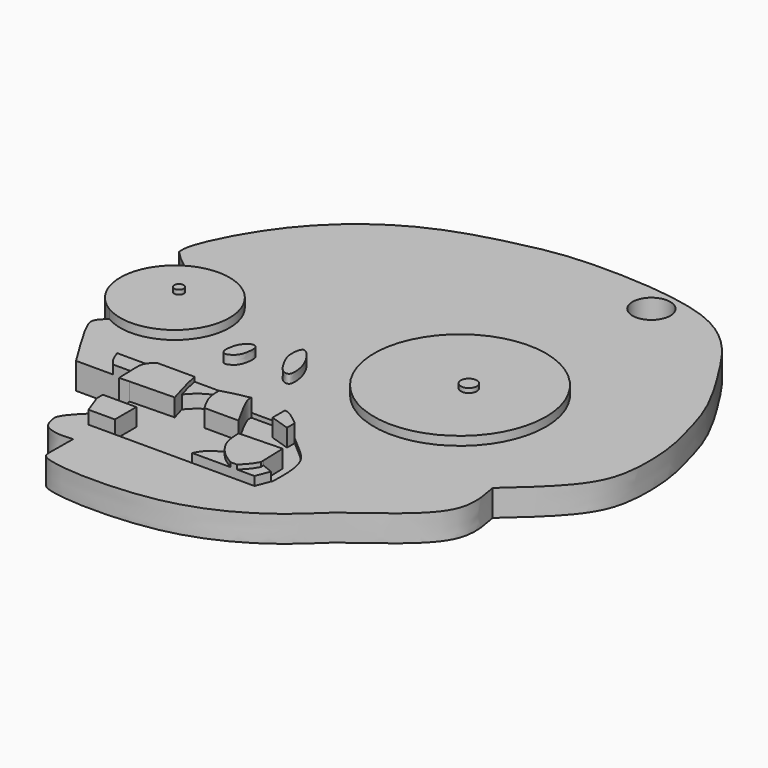
from build123d import *

# Parameters (mm, degrees)
F0_R     = 9.756
F0_R_2   = 2.14301661
F1_DEPTH = 3
F0_R_3   = 0.5489550531
F0_R_4   = 0.9110758453
F2_DEPTH = 4
F3_DEPTH = 4.5
F4_DEPTH = 4.5
F5_DEPTH = 2.5


# Not quite as in the source:
# - ends of sketch curves that miss each other by under 0.0002 mm in the source are joined


with BuildPart() as f1:
    # F0 (on Top) → F1 (new body)
    with BuildSketch(Plane.XY):
        with BuildLine():
            add(Edge.make_bspline(
                [(-1.2393802172, 30.2286203951), (-0.4158833716, 30.373480778), (1.6606665352, 30.7387642837), (7.9386116813, 30.9430876865), (18.147479825, 29.9352400746), (23.1024202655, 25.7119331789), (25.72137538, 21.6124660135), (29.4314571956, 15.6799496131), (30.7334478805, 10.40848904), (31.4866231448, 7.6721319387), (31.7667483963, 2.2460729415), (30.3960792989, -2.5468600017), (26.2945647642, -6.1923512069), (23.9523444325, -8.2741538063)],
                knots=[0, 0, 0, 0, 0.0633267686, 0.1596863377, 0.2826691674, 0.3774808941, 0.4616409818, 0.5634971311, 0.6515777447, 0.7163703966, 0.8033752015, 0.8877149899, 1, 1, 1, 1], degree=3))
            add(Edge.make_bspline(
                [(-1.2393802172, 30.2286203951), (-2.8705070942, 29.8823566818), (-6.4988427986, 29.112115561), (-14.107033655, 26.5390353225), (-22.1790734534, 19.7802047992), (-26.231732067, 11.4546819847), (-26.1231331955, 10.1430820977), (-26.0920431465, 9.7675928846)],
                knots=[0, 0, 0, 0, 0.1823196445, 0.4055581972, 0.6703764425, 0.9056342628, 1, 1, 1, 1], degree=3))
            add(Edge.make_bspline(
                [(-26.0920431465, 9.7675928846), (-25.7886867903, 9.446402666), (-25.0293246752, 8.6417283139), (-23.384300951, 7.4507044648), (-22.3954650109, 6.7330964966)],
                knots=[0, 0, 0, 0, 0.3993621606, 1, 1, 1, 1], degree=3))
            ThreePointArc((-22.3954650109, 6.7330964966), (-16.388075709, 6.4168152727), (-13.4720232753, 1.1551236967))
            ThreePointArc((-13.4720232753, 1.1551236967), (-16.6204187962, -4.2448565962), (-22.8706838798, -4.1650574556))
            add(Edge.make_bspline(
                [(-22.8706838798, -4.1650574556), (-23.2251432704, -4.503107188), (-23.8543858706, -5.1018227163), (-23.8274706305, -6.1029660819), (-22.5427366396, -8.3753891262), (-20.3011528826, -12.0943672024), (-20.1644091369, -12.2649352771), (-20.1410669833, -12.2940531)],
                knots=[0, 0, 0, 0, 0.1843482912, 0.3279717022, 0.5995926127, 0.9316769819, 1, 1, 1, 1], degree=3))
            Line((-20.1410669833, -12.2940531), (-15.9410070627, -12.2940531))
            add(Edge.make_bspline(
                [(-15.9410070627, -12.2940531), (-16.1547290947, -12.0513152103), (-16.6081258621, -11.5363632725), (-16.8757984305, -10.7686429845), (-17.0172955841, -10.3628104553)],
                knots=[0, 0, 0, 0, 0.4713796997, 1, 1, 1, 1], degree=3))
            Line((-17.0172955841, -10.3628104553), (-12.5004155561, -10.3628104553))
            Line((-12.5004155561, -10.3628104553), (-8.2129081711, -10.3628104553))
            Line((-8.2129081711, -10.3628104553), (-1.7728252569, -10.3628104553))
            Line((-1.7728252569, -10.3628104553), (1.3264130102, -10.3628104553))
            add(Edge.make_bspline(
                [(1.3264130102, -10.3628104553), (1.5699030442, -10.3549216682), (1.8133930781, -10.3470328812), (2.068254631, -10.389211361)],
                knots=[0, 0, 0, 0, 0.2797726741, 0.2797726741, 0.2797726741, 0.2797726741], degree=3))
            add(Edge.make_bspline(
                [(2.068254631, -10.389211361), (2.1914664058, -10.4096023744), (2.8617166916, -10.580494915), (3.6437610552, -11.2436017254), (4.2789415456, -11.7821805179)],
                knots=[0.2797726741, 0.2797726741, 0.2797726741, 0.2797726741, 0.4150276285, 1, 1, 1, 1], degree=3))
            add(Edge.make_bspline(
                [(4.2789415456, -11.7821805179), (4.6829303138, -12.1450168981), (5.5999948022, -12.9686644486), (8.0560238989, -14.8958762571), (7.9619883229, -17.9183800715), (7.9091731459, -19.6159724146)],
                knots=[0, 0, 0, 0, 0.2565884637, 0.5824621541, 1, 1, 1, 1], degree=3))
            add(Edge.make_bspline(
                [(7.8397894075, -19.5867830955), (7.8639386907, -19.5968842625), (7.8865559183, -19.6064283386), (7.9091731459, -19.6159724146)],
                knots=[0.8931074225, 0.8931074225, 0.8931074225, 0.8931074225, 1, 1, 1, 1], degree=3))
            add(Edge.make_bspline(
                [(7.2210850194, -21.1771205068), (7.4273304113, -20.6469827043), (7.6335758032, -20.1168449019), (7.8397894075, -19.5867830955)],
                knots=[0, 0, 0, 0, 1.7065313537, 1.7065313537, 1.7065313537, 1.7065313537], degree=3))
            Line((7.2210850194, -21.1771205068), (5.2385437302, -21.1771205068))
            Line((5.2385437302, -21.1771205068), (4.5115393586, -21.1771205068))
            Line((4.5115393586, -21.1771205068), (0.1495117176, -21.1771205068))
            Line((0.1495117176, -21.1771205068), (-8.6269685999, -21.1771205068))
            Line((-8.6269685999, -21.1771205068), (-11.6212656721, -21.1771205068))
            Line((-11.6212656721, -21.1771205068), (-12.4197443947, -18.9932379872))
            Line((-12.4197443947, -18.9932379872), (-12.5852758065, -19.1398113966))
            add(Edge.make_bspline(
                [(-10.952696187, -24.1973703964), (-11.6003607025, -24.2475742409), (-12.8304027144, -24.3429211934), (-14.4581285949, -23.7254439522), (-14.6736070417, -22.6233199395), (-15.038550408, -21.5870552272), (-13.5615867359, -20.1137223062), (-12.5852758065, -19.1398113966)],
                knots=[0, 0, 0, 0, 0.2162457448, 0.4106931052, 0.5661826538, 0.7132355897, 1, 1, 1, 1], degree=3))
            add(Edge.make_bspline(
                [(23.9523444325, -8.2741538063), (24.2863039744, -9.9748611419), (25.0090136589, -13.6552999598), (19.3340818803, -18.3065983827), (15.7324066153, -20.7445567564), (13.2149854072, -23.5297131407), (4.0834935552, -29.8946094699), (-10.9302506494, -29.1906042728), (-11.0010002399, -27.4544620035), (-10.9523846246, -24.5344095892), (-10.9525207478, -24.2320520286), (-10.952696187, -24.1973703964)],
                knots=[0, 0, 0, 0, 0.1169433124, 0.2530727642, 0.3618233297, 0.4588114113, 0.6358882656, 0.8281973553, 0.8861964274, 0.976190375, 0.9925215819, 0.9925215819, 0.9925215819, 0.9925215819], degree=3))
        make_face()
        with BuildLine():
            add(Edge.make_bspline(
                [(-9.6221137792, -2.3781536147), (-9.4655224083, -2.0993212718), (-9.0208657927, -1.6374110115), (-8.5262366968, -1.4918482785), (-8.0548862611, -1.7768664904), (-8.0508374383, -2.8141169089), (-8.3507435947, -3.8951758217), (-9.0186010158, -4.4028924818), (-9.7088724417, -4.5819747824), (-9.9941823947, -3.9236958827), (-9.8756994925, -3.1639822237), (-9.7687938604, -2.6393375514), (-9.6221137792, -2.3781536147)],
                knots=[0, 0, 0, 0, 0.1138345197, 0.1934305742, 0.2698157261, 0.3849908147, 0.5088302527, 0.6140567508, 0.7027480415, 0.7907303024, 0.8933705191, 1, 1, 1, 1], degree=3))
        make_face(mode=Mode.SUBTRACT)
        with BuildLine():
            add(Edge.make_bspline(
                [(-4.581714049, 0.4414755676), (-4.3886019619, 0.556001698), (-3.6219717469, -0.0557970156), (-2.5850360287, -1.81802008), (-2.4065766969, -3.5191596454), (-2.627381433, -4.0742860536), (-3.5558163843, -3.9967136296), (-4.6097436694, -2.0631900411), (-4.9778002041, -1.0265364593), (-4.8177214639, 0.3015101394), (-4.581714049, 0.4414755676)],
                knots=[0, 0, 0, 0, 0.1053234474, 0.2714857478, 0.4152922703, 0.4898158762, 0.5821472357, 0.743142993, 0.8712814152, 1, 1, 1, 1], degree=3))
        make_face(mode=Mode.SUBTRACT)
        with Locations((10.5493292212, 3.8432257716)):
            Circle(F0_R, mode=Mode.SUBTRACT)
        with Locations((13.4515836835, 27.3811984807)):
            Circle(F0_R_2, mode=Mode.SUBTRACT)
    extrude(amount=F1_DEPTH)

    # F0 (on Top) → F2 (join)
    with BuildSketch(Plane.XY):
        with BuildLine():
            add(Edge.make_bspline(
                [(-15.9410070627, -12.2940531), (-16.1547290947, -12.0513152103), (-16.6081258621, -11.5363632725), (-16.8757984305, -10.7686429845), (-17.0172955841, -10.3628104553)],
                knots=[0, 0, 0, 0, 0.4713796997, 1, 1, 1, 1], degree=3))
            Line((-15.9410070627, -12.2940531), (-13.3990075059, -12.2940531))
            add(Edge.make_bspline(
                [(-12.5004155561, -10.3628104553), (-12.8042925116, -10.6364223183), (-13.3531482467, -11.1306139227), (-13.4030830888, -11.8825646099), (-13.3990075059, -12.2940531)],
                knots=[0, 0, 0, 0, 0.2822962739, 0.5098771923, 0.5098771923, 0.5098771923, 0.5098771923], degree=3))
            Line((-12.5004155561, -10.3628104553), (-17.0172955841, -10.3628104553))
        make_face()
        with BuildLine():
            Line((-1.7728252569, -10.3628104553), (-8.2129081711, -10.3628104553))
            add(Edge.make_bspline(
                [(-8.2129081711, -10.3628104553), (-8.1550609219, -10.7006143743), (-8.0476180243, -11.3280362889), (-7.747571442, -12.4158381016), (-7.5893943801, -12.9649978611)],
                knots=[0, 0, 0, 0, 0.3777900329, 0.7016903371, 0.7016903371, 0.7016903371, 0.7016903371], degree=3))
            add(Edge.make_bspline(
                [(-7.5893943801, -12.9649978611), (-7.1117267836, -12.4364258807), (-6.4364554435, -11.6928519992), (-5.2333924432, -11.2084781414), (-4.8551141513, -11.0839256667)],
                knots=[0, 0, 0, 0, 0.4202161524, 0.5907091248, 0.5907091248, 0.5907091248, 0.5907091248], degree=3))
            add(Edge.make_bspline(
                [(-4.8551141513, -11.0839256667), (-3.9470072013, -10.7849210176), (-2.8599860204, -10.5738001088), (-1.7728252569, -10.3628104553)],
                knots=[0.5907091248, 0.5907091248, 0.5907091248, 0.5907091248, 1, 1, 1, 1], degree=3))
        make_face()
        with BuildLine():
            add(Edge.make_bspline(
                [(2.2680953621, -19.1644323351), (1.7322527396, -19.4720374585), (0.7474409463, -20.0374812634), (0.3369805018, -20.819646162), (0.1495117176, -21.1771205068)],
                knots=[0, 0, 0, 0, 0.5430655229, 1, 1, 1, 1], degree=3))
            Line((0.1495117176, -21.1771205068), (4.5115393586, -21.1771205068))
            add(Edge.make_bspline(
                [(2.2680953621, -19.1644323351), (2.5004401266, -19.5374508957), (3.2173678001, -20.3983675028), (4.0257518369, -20.8848033952), (4.5115393586, -21.1771205068)],
                knots=[0.4760539781, 0.4760539781, 0.4760539781, 0.4760539781, 0.6851416803, 1, 1, 1, 1], degree=3))
        make_face()
        with BuildLine():
            add(Edge.make_bspline(
                [(6.5981289918, -19.4641191504), (6.4561431042, -19.7211838775), (6.1459175946, -20.2828455842), (5.5575977759, -20.8626723579), (5.2385437302, -21.1771205068)],
                knots=[0, 0, 0, 0, 0.4576860484, 1, 1, 1, 1], degree=3))
            Line((5.2385437302, -21.1771205068), (7.2210850194, -21.1771205068))
            add(Edge.make_bspline(
                [(7.2210850194, -21.1771205068), (7.4273304113, -20.6469827043), (7.6335758032, -20.1168449019), (7.8398211952, -19.5867070995)],
                knots=[0, 0, 0, 0, 1.7065313537, 1.7065313537, 1.7065313537, 1.7065313537], degree=3))
            add(Edge.make_bspline(
                [(6.5868723652, -19.0981086926), (7.0054958994, -19.2586307437), (7.5616668588, -19.4718956366), (7.7898889474, -19.5659107211), (7.8398211952, -19.5867070995)],
                knots=[0, 0, 0, 0, 0.6722317651, 0.8931074225, 0.8931074225, 0.8931074225, 0.8931074225], degree=3))
            Line((6.5868723652, -19.0981086926), (6.5981289918, -19.4641191504))
        make_face()
        with BuildLine():
            ThreePointArc((-13.4720232753, 1.1551236967), (-16.388075709, 6.4168152727), (-22.3954650109, 6.7330964966))
            ThreePointArc((-22.3954650109, 6.7330964966), (-25.8763207665, 1.4254427244), (-22.8706838798, -4.1650574556))
            ThreePointArc((-22.8706838798, -4.1650574556), (-16.6204187962, -4.2448565962), (-13.4720232753, 1.1551236967))
        make_face()
        with Locations((-20.0864113867, 2.2520758212)):
            Circle(F0_R_3, mode=Mode.SUBTRACT)
        with Locations((10.5493292212, 3.8432257716)):
            Circle(F0_R)
        with Locations((11.5533228964, 3.8432257716)):
            Circle(F0_R_4, mode=Mode.SUBTRACT)
        with BuildLine():
            add(Edge.make_bspline(
                [(-4.581714049, 0.4414755676), (-4.3886019619, 0.556001698), (-3.6219717469, -0.0557970156), (-2.5850360287, -1.81802008), (-2.4065766969, -3.5191596454), (-2.627381433, -4.0742860536), (-3.5558163843, -3.9967136296), (-4.6097436694, -2.0631900411), (-4.9778002041, -1.0265364593), (-4.8177214639, 0.3015101394), (-4.581714049, 0.4414755676)],
                knots=[0, 0, 0, 0, 0.1053234474, 0.2714857478, 0.4152922703, 0.4898158762, 0.5821472357, 0.743142993, 0.8712814152, 1, 1, 1, 1], degree=3))
        make_face()
        with BuildLine():
            add(Edge.make_bspline(
                [(-9.6221137792, -2.3781536147), (-9.4655224083, -2.0993212718), (-9.0208657927, -1.6374110115), (-8.5262366968, -1.4918482785), (-8.0548862611, -1.7768664904), (-8.0508374383, -2.8141169089), (-8.3507435947, -3.8951758217), (-9.0186010158, -4.4028924818), (-9.7088724417, -4.5819747824), (-9.9941823947, -3.9236958827), (-9.8756994925, -3.1639822237), (-9.7687938604, -2.6393375514), (-9.6221137792, -2.3781536147)],
                knots=[0, 0, 0, 0, 0.1138345197, 0.1934305742, 0.2698157261, 0.3849908147, 0.5088302527, 0.6140567508, 0.7027480415, 0.7907303024, 0.8933705191, 1, 1, 1, 1], degree=3))
        make_face()
    extrude(amount=F2_DEPTH)

    # F0 (on Top) → F3 (join)
    with BuildSketch(Plane.XY):
        with BuildLine():
            add(Edge.make_bspline(
                [(-12.5004155561, -10.3628104553), (-12.8042925116, -10.6364223183), (-13.3531482467, -11.1306139227), (-13.4030830888, -11.8825646099), (-13.3990075059, -12.2940531)],
                knots=[0, 0, 0, 0, 0.2822962739, 0.5098771923, 0.5098771923, 0.5098771923, 0.5098771923], degree=3))
            add(Edge.make_bspline(
                [(-13.3990075059, -12.2940531), (-13.3970104097, -12.4956885818), (-13.3629923661, -13.3937925117), (-13.367018161, -14.7388380525), (-13.3004729779, -14.7062276033), (-13.2943978533, -14.7032504901)],
                knots=[0.5098771923, 0.5098771923, 0.5098771923, 0.5098771923, 0.6213952279, 0.9654359482, 1, 1, 1, 1], degree=3))
            Line((-13.2943978533, -14.7032504901), (-12.1538676941, -14.6771812873))
            Line((-12.1538676941, -14.6771812873), (-7.1189762093, -14.5620983094))
            add(Edge.make_bspline(
                [(-7.5893943801, -12.9649978611), (-7.4437145355, -13.4707697319), (-7.2813453724, -14.0164340206), (-7.1189762093, -14.5620983094)],
                knots=[0.7016903371, 0.7016903371, 0.7016903371, 0.7016903371, 1, 1, 1, 1], degree=3))
            add(Edge.make_bspline(
                [(-8.2129081711, -10.3628104553), (-8.1550609219, -10.7006143743), (-8.0476180243, -11.3280362889), (-7.747571442, -12.4158381016), (-7.5893943801, -12.9649978611)],
                knots=[0, 0, 0, 0, 0.3777900329, 0.7016903371, 0.7016903371, 0.7016903371, 0.7016903371], degree=3))
            Line((-8.2129081711, -10.3628104553), (-12.5004155561, -10.3628104553))
        make_face()
        with BuildLine():
            add(Edge.make_bspline(
                [(-1.7728252569, -10.3628104553), (-1.7983770554, -10.4823579011), (-1.9012496825, -10.9636610001), (-0.7616136008, -13.0064418165), (0.0949563982, -14.5418308675)],
                knots=[0, 0, 0, 0, 0.2483828717, 1, 1, 1, 1], degree=3))
            add(Edge.make_bspline(
                [(-4.8551141513, -11.0839256667), (-3.9470072013, -10.7849210176), (-2.8599860204, -10.5738001088), (-1.7728252569, -10.3628104553)],
                knots=[0.5907091248, 0.5907091248, 0.5907091248, 0.5907091248, 1, 1, 1, 1], degree=3))
            add(Edge.make_bspline(
                [(-4.8551141513, -11.0839256667), (-4.8562759886, -11.57887424), (-4.8557941721, -12.6637126662), (-4.1750627603, -13.853987798), (-3.807129804, -14.4973201677)],
                knots=[0, 0, 0, 0, 0.459545709, 1, 1, 1, 1], degree=3))
            Line((-3.807129804, -14.4973201677), (0, -14.4973201677))
            Line((0, -14.4973201677), (0.0949563982, -14.5418308675))
        make_face()
        with BuildLine():
            add(Edge.make_bspline(
                [(2.068254631, -10.389211361), (2.1914664058, -10.4096023744), (2.8617166916, -10.580494915), (3.6437610552, -11.2436017254), (4.2789415456, -11.7821805179)],
                knots=[0.2797726741, 0.2797726741, 0.2797726741, 0.2797726741, 0.4150276285, 1, 1, 1, 1], degree=3))
            Line((2.068254631, -10.389211361), (2.068254631, -10.6616893224))
            Line((2.068254631, -10.6616893224), (2.068254631, -12.1679380536))
            Line((2.068254631, -12.1679380536), (4.2789415456, -12.8801064566))
            Line((4.2789415456, -12.8801064566), (4.2789415456, -11.7821805179))
        make_face()
        with BuildLine():
            add(Edge.make_bspline(
                [(2.2680953621, -19.1644323351), (2.5004401266, -19.5374508957), (3.2173678001, -20.3983675028), (4.0257518369, -20.8848033952), (4.5115393586, -21.1771205068)],
                knots=[0.4760539781, 0.4760539781, 0.4760539781, 0.4760539781, 0.6851416803, 1, 1, 1, 1], degree=3))
            Line((4.5115393586, -21.1771205068), (5.2385437302, -21.1771205068))
            add(Edge.make_bspline(
                [(6.5981289918, -19.4641191504), (6.4561431042, -19.7211838775), (6.1459175946, -20.2828455842), (5.5575977759, -20.8626723579), (5.2385437302, -21.1771205068)],
                knots=[0, 0, 0, 0, 0.4576860484, 1, 1, 1, 1], degree=3))
            Line((6.5981289918, -19.4641191504), (6.5868723652, -19.0981086926))
            Line((6.5868723652, -19.0981086926), (6.4996741712, -16.2628497928))
            Line((6.4996741712, -16.2628497928), (1.6102727968, -16.4132229984))
            add(Edge.make_bspline(
                [(1.6102727968, -16.4132229984), (1.6331093101, -17.0782850727), (1.6654605521, -18.0204422193), (2.1125109599, -18.9146489157), (2.2680953621, -19.1644323351)],
                knots=[0, 0, 0, 0, 0.3360431403, 0.4760539781, 0.4760539781, 0.4760539781, 0.4760539781], degree=3))
        make_face()
        Polygon((-12.4197443947, -18.1323774159), (-12.4197443947, -18.9932379872), (-11.6212656721, -21.1771205068), (-8.6269685999, -21.1771205068), (-8.6269685999, -18.1323774159), (-11.7639265954, -18.1323774159), align=None)
    extrude(amount=F3_DEPTH)

    # F0 (on Top) → F4 (join)
    with BuildSketch(Plane.XY):
        with Locations((-20.0864113867, 2.2520758212)):
            Circle(F0_R_3)
        with Locations((11.5533228964, 3.8432257716)):
            Circle(F0_R_4)
    extrude(amount=F4_DEPTH)

    # F0 (on Top) → F5 (join)
    with BuildSketch(Plane.XY):
        with BuildLine():
            Line((-11.7639265954, -17.8953260183), (-11.7639265954, -18.1323774159))
            Line((-11.7639265954, -18.1323774159), (-8.6269685999, -18.1323774159))
            Line((-8.6269685999, -18.1323774159), (-8.6269685999, -21.1771205068))
            Line((-8.6269685999, -21.1771205068), (0.1495117176, -21.1771205068))
            add(Edge.make_bspline(
                [(2.2680953621, -19.1644323351), (1.7322527396, -19.4720374585), (0.7474409463, -20.0374812634), (0.3369805018, -20.819646162), (0.1495117176, -21.1771205068)],
                knots=[0, 0, 0, 0, 0.5430655229, 1, 1, 1, 1], degree=3))
            add(Edge.make_bspline(
                [(1.6102727968, -16.4132229984), (1.6331093101, -17.0782850727), (1.6654605521, -18.0204422193), (2.1125109599, -18.9146489157), (2.2680953621, -19.1644323351)],
                knots=[0, 0, 0, 0, 0.3360431403, 0.4760539781, 0.4760539781, 0.4760539781, 0.4760539781], degree=3))
            Line((1.6102727968, -16.4132229984), (6.4996741712, -16.2628497928))
            Line((6.4996741712, -16.2628497928), (6.5868723652, -19.0981086926))
            add(Edge.make_bspline(
                [(6.5868723652, -19.0981086926), (7.0054958994, -19.2586307437), (7.5616668588, -19.4718956366), (7.7898889474, -19.5659107211), (7.8397894075, -19.5867830955)],
                knots=[0, 0, 0, 0, 0.6722317651, 0.8931074225, 0.8931074225, 0.8931074225, 0.8931074225], degree=3))
            add(Edge.make_bspline(
                [(7.8397894075, -19.5867830955), (7.8639386907, -19.5968842625), (7.8865559183, -19.6064283386), (7.9091731459, -19.6159724146)],
                knots=[0.8931074225, 0.8931074225, 0.8931074225, 0.8931074225, 1, 1, 1, 1], degree=3))
            add(Edge.make_bspline(
                [(4.2789415456, -11.7821805179), (4.6829303138, -12.1450168981), (5.5999948022, -12.9686644486), (8.0560238989, -14.8958762571), (7.9619883229, -17.9183800715), (7.9091731459, -19.6159724146)],
                knots=[0, 0, 0, 0, 0.2565884637, 0.5824621541, 1, 1, 1, 1], degree=3))
            Line((4.2789415456, -11.7821805179), (4.2789415456, -12.8801064566))
            Line((4.2789415456, -12.8801064566), (2.068254631, -12.1679380536))
            Line((2.068254631, -12.1679380536), (2.068254631, -10.6616893224))
            Line((2.068254631, -10.6616893224), (2.068254631, -10.389211361))
            add(Edge.make_bspline(
                [(1.3264130102, -10.3628104553), (1.5699030442, -10.3549216682), (1.8133930781, -10.3470328812), (2.068254631, -10.389211361)],
                knots=[0, 0, 0, 0, 0.2797726741, 0.2797726741, 0.2797726741, 0.2797726741], degree=3))
            Line((1.3264130102, -10.3628104553), (-1.7728252569, -10.3628104553))
            add(Edge.make_bspline(
                [(-1.7728252569, -10.3628104553), (-1.7983770554, -10.4823579011), (-1.9012496825, -10.9636610001), (-0.7616136008, -13.0064418165), (0.0949563982, -14.5418308675)],
                knots=[0, 0, 0, 0, 0.2483828717, 1, 1, 1, 1], degree=3))
            Line((0.0949563982, -14.5418308675), (0, -14.4973201677))
            Line((0, -14.4973201677), (-3.807129804, -14.4973201677))
            add(Edge.make_bspline(
                [(-4.8551141513, -11.0839256667), (-4.8562759886, -11.57887424), (-4.8557941721, -12.6637126662), (-4.1750627603, -13.853987798), (-3.807129804, -14.4973201677)],
                knots=[0, 0, 0, 0, 0.459545709, 1, 1, 1, 1], degree=3))
            add(Edge.make_bspline(
                [(-7.5893943801, -12.9649978611), (-7.1117267836, -12.4364258807), (-6.4364554435, -11.6928519992), (-5.2333924432, -11.2084781414), (-4.8551141513, -11.0839256667)],
                knots=[0, 0, 0, 0, 0.4202161524, 0.5907091248, 0.5907091248, 0.5907091248, 0.5907091248], degree=3))
            add(Edge.make_bspline(
                [(-7.5893943801, -12.9649978611), (-7.4437145355, -13.4707697319), (-7.2813453724, -14.0164340206), (-7.1189762093, -14.5620983094)],
                knots=[0.7016903371, 0.7016903371, 0.7016903371, 0.7016903371, 1, 1, 1, 1], degree=3))
            Line((-7.1189762093, -14.5620983094), (-12.1538676941, -14.6771812873))
            add(Edge.make_bspline(
                [(-12.1538676941, -14.6771812873), (-12.0238873279, -15.7498961977), (-11.8939069617, -16.822611108), (-11.7639265954, -17.8953260183)],
                knots=[0, 0, 0, 0, 3.2416831384, 3.2416831384, 3.2416831384, 3.2416831384], degree=3))
        make_face()
    extrude(amount=F5_DEPTH)


solid = f1.part
